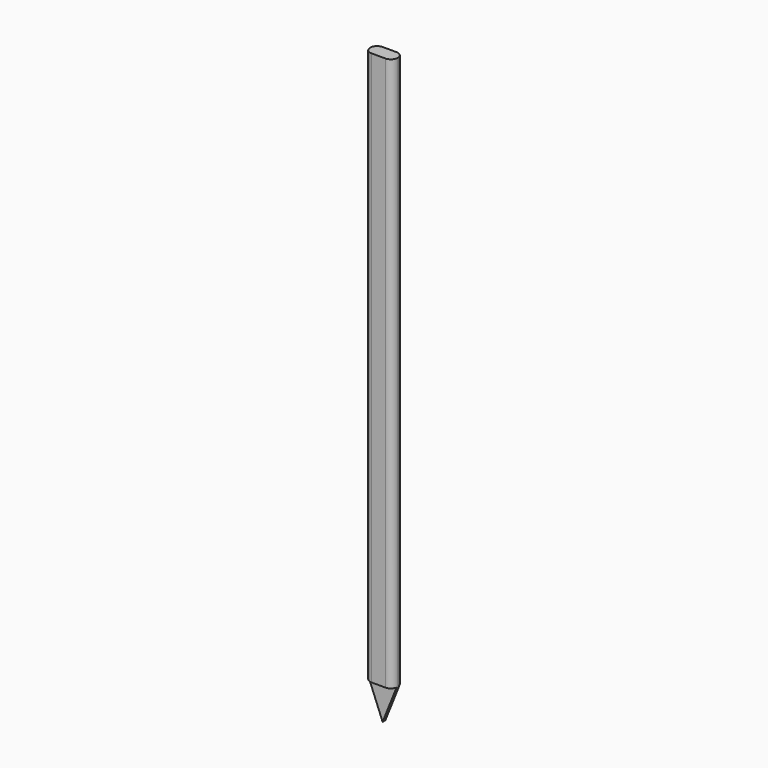
from build123d import *

# Parameters (mm, degrees)
F0_W     = 40
F0_H     = 20
F1_DEPTH = 800
F2_R     = 9.99999
F4_DEPTH = 2.5


# Not quite as in the source:
# - a fillet or chamfer is up to 0.001 mm smaller than in the source, because OpenCascade refuses the exact size


with BuildPart() as f1:
    # F0 (on Top) → F1 (new body)
    with BuildSketch(Plane.XY):
        Rectangle(F0_W, F0_H)
    extrude(amount=F1_DEPTH)

    # F2 (radius 10 in the source; OpenCascade refuses exactly that, so slightly less here)
    f2_edges = [f1.edges().sort_by_distance(p)[0] for p in [
        (20, -10, 400),
        (20, 10, 400),
        (-20, -10, 400),
        (-20, 10, 400),
    ]]
    fillet(f2_edges, radius=F2_R)

    # F3 (on Front) → F4 (join, symmetric)
    with BuildSketch(Plane.XZ):
        Polygon((19.9430335092, 0), (-20.0569664908, 0), (0, -50), align=None)
    extrude(amount=F4_DEPTH, both=True)


solid = f1.part
